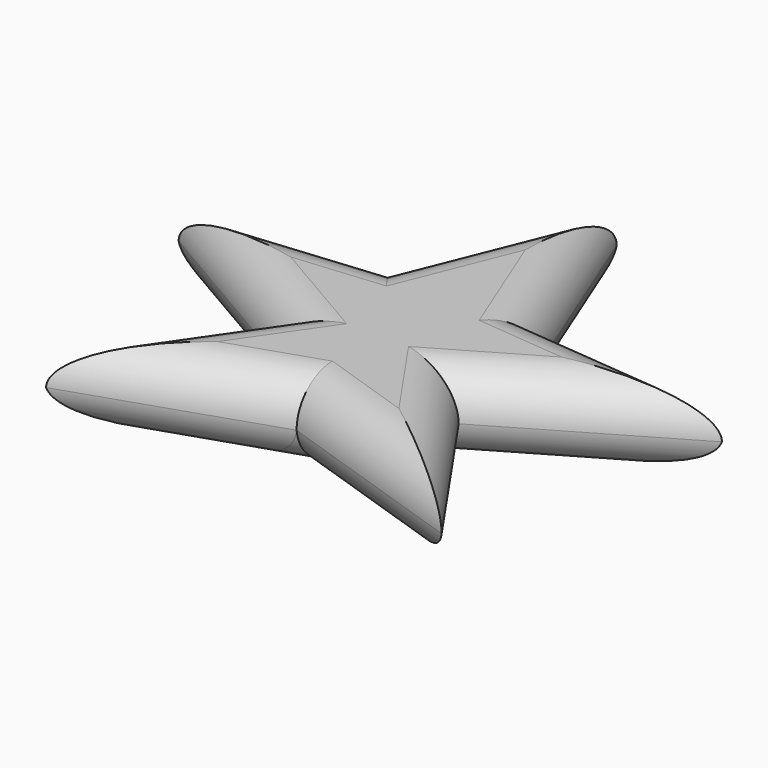
from build123d import *

# Parameters (mm, degrees)
F1_DEPTH      = 9.652
F2_R          = 5.08
F3_T4_DEPTH   = 48.7182027165
F3_T9_DEPTH   = 49.6907337444
F3_T14_DEPTH  = 49.6907337444
F3_T19_DEPTH  = 48.7182027165
F3_T24_DEPTH  = 50.0877618637
F3_T29_DEPTH  = 47.5225066811
F3_T34_DEPTH  = 50.1646809025
F3_T39_DEPTH  = 50.1646809025
F3_T44_DEPTH  = 47.5225066811
F3_T49_DEPTH  = 50.0877618637
F3_T55_DEPTH  = 49.6907337444
F3_T59_DEPTH  = 48.7182027165
F3_T66_DEPTH  = 49.6907337444
F3_T70_DEPTH  = 48.7182027165
F3_T77_DEPTH  = 50.0877618637
F3_T81_DEPTH  = 47.5225066811
F3_T88_DEPTH  = 50.1646809025
F3_T92_DEPTH  = 50.1646809025
F3_T99_DEPTH  = 47.5225066811
F3_T103_DEPTH = 50.0877618637


# Not quite as in the source:
# - a fillet or chamfer that OpenCascade refuses, or shapes differently, is made with other operations: its cross-section is extruded or revolved along the edge and cut away or added


with BuildPart() as f1:
    # F0 (on Top) → F1 (new body)
    with BuildSketch(Plane.XY):
        Polygon((9.0920295568, 17.9841070124), (0, 40.6463289496), (-9.0920295568, 17.9841070124), (-32.4367642404, 15.8125049123), (-10.9921818601, 3.3257867829), (-23.6146248879, -14.9971136204), (0, -7.1255727671), (23.6146248879, -14.9971136204), (10.9921818601, 3.3257867829), (32.4367642404, 15.8125049123), align=None)
    extrude(amount=F1_DEPTH)

    # F2
    f2_edges = [f1.edges().sort_by_distance(p)[0] for p in [
        (21.714473, 9.569146, 9.652),
        (17.303403, -5.835663, 9.652),
        (11.807312, -11.061343, 9.652),
        (-11.807312, -11.061343, 9.652),
        (-17.303403, -5.835663, 9.652),
        (-21.714473, 9.569146, 9.652),
        (-4.546015, 29.315218, 9.652),
        (4.546015, 29.315218, 9.652),
        (20.764397, 16.898306, 9.652),
        (-20.764397, 16.898306, 9.652),
    ]]
    fillet(f2_edges, radius=F2_R)

    # F3: fillet of radius 5.08 on 10 edges, made by hand


with BuildPart() as f3_tool2:
    # F3_s3 → F3_t4 (new body)
    with BuildSketch(Plane(origin=(43.2821955638, -4.026248662, 0), x_dir=(0, 0, 1), z_dir=(-0.9957012204, 0.0926233213, 0))):
        with BuildLine():
            ThreePointArc((4.572, 18.7489312754), (1.3125711686, 17.1021626927), (0, 13.6943950949))
            Line((0, 13.6943950949), (-0.1016, 13.6943950949))
            Line((-0.1016, 13.6943950949), (-0.1016, 18.7489312754))
            Line((-0.1016, 18.7489312754), (0, 18.8505312754))
            ThreePointArc((0, 18.8505312754), (2.286, 18.8505312754), (4.56184, 18.8500219991))
            Line((4.56184, 18.8500219991), (4.572, 18.7489312754))
        make_face()
    extrude(amount=F3_T4_DEPTH)

    split(bisect_by=Plane(origin=(14.046321235, 5.6353506813, 0), x_dir=(0, 0, 1), z_dir=(0.928092919, 0.3723486723, 0)), keep=Keep.TOP)


with BuildPart() as f1_1:
    add(f1.part)

    # F3_t1: cut F3_tool2
    add(f3_tool2.part, mode=Mode.SUBTRACT)


with BuildPart() as f3_tool7:
    # F3_s8 → F3_t9 (new body)
    with BuildSketch(Plane(origin=(-0.2491670879, 0.6210582369, 0), x_dir=(0, 0, 1), z_dir=(-0.3723486723, 0.928092919, 0))):
        with BuildLine():
            ThreePointArc((4.572, 15.1346066199), (1.3125711686, 13.4878380371), (0, 10.0800704394))
            Line((0, 10.0800704394), (-0.1016, 10.0800704394))
            Line((-0.1016, 10.0800704394), (-0.1016, 15.1346066199))
            Line((-0.1016, 15.1346066199), (0, 15.2362066199))
            ThreePointArc((0, 15.2362066199), (2.286, 15.2362066199), (4.56184, 15.2356973435))
            Line((4.56184, 15.2356973435), (4.572, 15.1346066199))
        make_face()
    extrude(amount=F3_T9_DEPTH)

    split(bisect_by=Plane(origin=(1.7365882856, 18.6683337526, 0), x_dir=(0, 0, 1), z_dir=(0.0926233213, 0.9957012204, 0)), keep=Keep.TOP)


with BuildPart() as f1_2:
    add(f1_1.part)

    # F3_t6: cut F3_tool7
    add(f3_tool7.part, mode=Mode.SUBTRACT)


with BuildPart() as f3_tool12:
    # F3_s13 → F3_t14 (new body)
    with BuildSketch(Plane(origin=(18.7514458253, 46.7386763625, 0), x_dir=(0, 0, 1), z_dir=(-0.3723486723, -0.928092919, 0))):
        with BuildLine():
            ThreePointArc((0, 10.0800704394), (1.3125711686, 13.4878380371), (4.572, 15.1346066199))
            Line((4.572, 15.1346066199), (4.56184, 15.2356973435))
            ThreePointArc((4.56184, 15.2356973435), (2.286, 15.2362066199), (0, 15.2362066199))
            Line((0, 15.2362066199), (-0.1016, 15.1346066199))
            Line((-0.1016, 15.1346066199), (-0.1016, 10.0800704394))
            Line((-0.1016, 10.0800704394), (0, 10.0800704394))
        make_face()
    extrude(amount=F3_T14_DEPTH)

    split(bisect_by=Plane(origin=(-1.7365882856, 18.6683337526, 0), x_dir=(0, 0, 1), z_dir=(-0.0926233213, 0.9957012204, 0)), keep=Keep.TOP)


with BuildPart() as f1_3:
    add(f1_2.part)

    # F3_t11: cut F3_tool12
    add(f3_tool12.part, mode=Mode.SUBTRACT)


with BuildPart() as f3_tool17:
    # F3_s18 → F3_t19 (new body)
    with BuildSketch(Plane(origin=(5.2265783378, 0.4861930816, 0), x_dir=(0, 0, 1), z_dir=(-0.9957012204, -0.0926233213, 0))):
        with BuildLine():
            ThreePointArc((0, 13.6943950949), (1.3125711686, 17.1021626927), (4.572, 18.7489312754))
            Line((4.572, 18.7489312754), (4.56184, 18.8500219991))
            ThreePointArc((4.56184, 18.8500219991), (2.286, 18.8505312754), (0, 18.8505312754))
            Line((0, 18.8505312754), (-0.1016, 18.7489312754))
            Line((-0.1016, 18.7489312754), (-0.1016, 13.6943950949))
            Line((-0.1016, 13.6943950949), (0, 13.6943950949))
        make_face()
    extrude(amount=F3_T19_DEPTH)

    split(bisect_by=Plane(origin=(-14.046321235, 5.6353506813, 0), x_dir=(0, 0, 1), z_dir=(-0.928092919, 0.3723486723, 0)), keep=Keep.TOP)


with BuildPart() as f1_4:
    add(f1_3.part)

    # F3_t16: cut F3_tool17
    add(f3_tool17.part, mode=Mode.SUBTRACT)


with BuildPart() as f3_tool22:
    # F3_s23 → F3_t24 (new body)
    with BuildSketch(Plane(origin=(-42.019750379, 24.4671950025, 0), x_dir=(0, 0, 1), z_dir=(0.8641753945, -0.5031907068, 0))):
        with BuildLine():
            ThreePointArc((0, -2.3974355258), (1.3125711686, 1.0103320719), (4.572, 2.6571006547))
            Line((4.572, 2.6571006547), (4.56184, 2.7581913783))
            ThreePointArc((4.56184, 2.7581913783), (2.286, 2.7587006547), (0, 2.7587006547))
            Line((0, 2.7587006547), (-0.1016, 2.6571006547))
            Line((-0.1016, 2.6571006547), (-0.1016, -2.3974355258))
            Line((-0.1016, -2.3974355258), (0, -2.3974355258))
        make_face()
    extrude(amount=F3_T24_DEPTH)

    split(bisect_by=Plane(origin=(-9.0082519421, 6.2056849307, 0), x_dir=(0, 0, 1), z_dir=(-0.8235075899, 0.5673052523, 0)), keep=Keep.TOP)


with BuildPart() as f1_5:
    add(f1_4.part)

    # F3_t21: cut F3_tool22
    add(f3_tool22.part, mode=Mode.SUBTRACT)


with BuildPart() as f3_tool27:
    # F3_s28 → F3_t29 (new body)
    with BuildSketch(Plane(origin=(5.1847323903, 7.5262241228, 0), x_dir=(0, 0, 1), z_dir=(-0.5673052523, -0.8235075899, 0))):
        with BuildLine():
            ThreePointArc((0, 5.8843453213), (1.3125711686, 9.292112919), (4.572, 10.9388815018))
            Line((4.572, 10.9388815018), (4.56184, 11.0399722254))
            ThreePointArc((4.56184, 11.0399722254), (2.286, 11.0404815018), (0, 11.0404815018))
            Line((0, 11.0404815018), (-0.1016, 10.9388815018))
            Line((-0.1016, 10.9388815018), (-0.1016, 5.8843453213))
            Line((-0.1016, 5.8843453213), (0, 5.8843453213))
        make_face()
    extrude(amount=F3_T29_DEPTH)

    split(bisect_by=Plane(origin=(-1.3370283566, -2.2962010066, 0), x_dir=(0, 0, 1), z_dir=(-0.5031907068, -0.8641753945, 0)), keep=Keep.TOP)


with BuildPart() as f1_6:
    add(f1_5.part)

    # F3_t26: cut F3_tool27
    add(f3_tool27.part, mode=Mode.SUBTRACT)


with BuildPart() as f3_tool32:
    # F3_s33 → F3_t34 (new body)
    with BuildSketch(Plane(origin=(-37.7401818022, -12.5800593605, 0), x_dir=(0, 0, 1), z_dir=(0.9486833074, 0.316227738, 0))):
        with BuildLine():
            ThreePointArc((0, 1.7053757593), (1.3125711686, 5.1131433571), (4.572, 6.7599119398))
            Line((4.572, 6.7599119398), (4.56184, 6.8610026635))
            ThreePointArc((4.56184, 6.8610026635), (2.286, 6.8615119398), (0, 6.8615119398))
            Line((0, 6.8615119398), (-0.1016, 6.7599119398))
            Line((-0.1016, 6.7599119398), (-0.1016, 1.7053757593))
            Line((-0.1016, 1.7053757593), (0, 1.7053757593))
        make_face()
    extrude(amount=F3_T34_DEPTH)

    split(bisect_by=Plane(origin=(-2.1376716615, -6.4130156168, 0), x_dir=(0, 0, 1), z_dir=(-0.316227738, -0.9486833074, 0)), keep=Keep.TOP)


with BuildPart() as f1_7:
    add(f1_6.part)

    # F3_t31: cut F3_tool32
    add(f3_tool32.part, mode=Mode.SUBTRACT)


with BuildPart() as f3_tool37:
    # F3_s38 → F3_t39 (new body)
    with BuildSketch(Plane(origin=(-9.8502135912, 3.2834042067, 0), x_dir=(0, 0, 1), z_dir=(0.9486833074, -0.316227738, 0))):
        with BuildLine():
            ThreePointArc((0, 1.7053757593), (1.3125711686, 5.1131433571), (4.572, 6.7599119398))
            Line((4.572, 6.7599119398), (4.56184, 6.8610026635))
            ThreePointArc((4.56184, 6.8610026635), (2.286, 6.8615119398), (0, 6.8615119398))
            Line((0, 6.8615119398), (-0.1016, 6.7599119398))
            Line((-0.1016, 6.7599119398), (-0.1016, 1.7053757593))
            Line((-0.1016, 1.7053757593), (0, 1.7053757593))
        make_face()
    extrude(amount=F3_T39_DEPTH)

    split(bisect_by=Plane(origin=(2.1376716615, -6.4130156168, 0), x_dir=(0, 0, 1), z_dir=(0.316227738, -0.9486833074, 0)), keep=Keep.TOP)


with BuildPart() as f1_8:
    add(f1_7.part)

    # F3_t36: cut F3_tool37
    add(f3_tool37.part, mode=Mode.SUBTRACT)


with BuildPart() as f3_tool42:
    # F3_s43 → F3_t44 (new body)
    with BuildSketch(Plane(origin=(21.7750352542, -31.6089208215, 0), x_dir=(0, 0, 1), z_dir=(-0.5673052523, 0.8235075899, 0))):
        with BuildLine():
            ThreePointArc((0, 5.8843453213), (1.3125711686, 9.292112919), (4.572, 10.9388815018))
            Line((4.572, 10.9388815018), (4.56184, 11.0399722254))
            ThreePointArc((4.56184, 11.0399722254), (2.286, 11.0404815018), (0, 11.0404815018))
            Line((0, 11.0404815018), (-0.1016, 10.9388815018))
            Line((-0.1016, 10.9388815018), (-0.1016, 5.8843453213))
            Line((-0.1016, 5.8843453213), (0, 5.8843453213))
        make_face()
    extrude(amount=F3_T44_DEPTH)

    split(bisect_by=Plane(origin=(1.3370283566, -2.2962010066, 0), x_dir=(0, 0, 1), z_dir=(0.5031907068, -0.8641753945, 0)), keep=Keep.TOP)


with BuildPart() as f1_9:
    add(f1_8.part)

    # F3_t41: cut F3_tool42
    add(f3_tool42.part, mode=Mode.SUBTRACT)


with BuildPart() as f3_tool47:
    # F3_s48 → F3_t49 (new body)
    with BuildSketch(Plane(origin=(-1.2648609916, -0.7365012941, 0), x_dir=(0, 0, 1), z_dir=(0.8641753945, 0.5031907068, 0))):
        with BuildLine():
            ThreePointArc((0, -2.3974355258), (1.3125711686, 1.0103320719), (4.572, 2.6571006547))
            Line((4.572, 2.6571006547), (4.56184, 2.7581913783))
            ThreePointArc((4.56184, 2.7581913783), (2.286, 2.7587006547), (0, 2.7587006547))
            Line((0, 2.7587006547), (-0.1016, 2.6571006547))
            Line((-0.1016, 2.6571006547), (-0.1016, -2.3974355258))
            Line((-0.1016, -2.3974355258), (0, -2.3974355258))
        make_face()
    extrude(amount=F3_T49_DEPTH)

    split(bisect_by=Plane(origin=(9.0082519421, 6.2056849307, 0), x_dir=(0, 0, 1), z_dir=(0.8235075899, 0.5673052523, 0)), keep=Keep.TOP)


with BuildPart() as f1_10:
    add(f1_9.part)

    # F3_t46: cut F3_tool47
    add(f3_tool47.part, mode=Mode.SUBTRACT)


with BuildPart() as f3_tool53:
    # F3_s54 → F3_t55 (new body)
    with BuildSketch(Plane(origin=(-0.2491670879, 0.6210582369, 0), x_dir=(0, 0, 1), z_dir=(-0.3723486723, 0.928092919, 0))):
        with BuildLine():
            ThreePointArc((4.572, 15.1346066199), (1.3125711686, 13.4878380371), (0, 10.0800704394))
            Line((0, 10.0800704394), (-0.1016, 10.0800704394))
            Line((-0.1016, 10.0800704394), (-0.1016, 15.1346066199))
            Line((-0.1016, 15.1346066199), (0, 15.2362066199))
            ThreePointArc((0, 15.2362066199), (2.286, 15.2362066199), (4.56184, 15.2356973435))
            Line((4.56184, 15.2356973435), (4.572, 15.1346066199))
        make_face()
    extrude(amount=F3_T55_DEPTH)

    split(bisect_by=Plane(origin=(1.7365882856, 18.6683337526, 0), x_dir=(0, 0, 1), z_dir=(-0.0926233213, -0.9957012204, 0)), keep=Keep.TOP)


with BuildPart() as f3_tool57:
    # F3_s58 → F3_t59 (new body)
    with BuildSketch(Plane(origin=(43.2821955638, -4.026248662, 0), x_dir=(0, 0, 1), z_dir=(-0.9957012204, 0.0926233213, 0))):
        with BuildLine():
            ThreePointArc((4.572, 18.7489312754), (1.3125711686, 17.1021626927), (0, 13.6943950949))
            Line((0, 13.6943950949), (-0.1016, 13.6943950949))
            Line((-0.1016, 13.6943950949), (-0.1016, 18.7489312754))
            Line((-0.1016, 18.7489312754), (0, 18.8505312754))
            ThreePointArc((0, 18.8505312754), (2.286, 18.8505312754), (4.56184, 18.8500219991))
            Line((4.56184, 18.8500219991), (4.572, 18.7489312754))
        make_face()
    extrude(amount=F3_T59_DEPTH)

    split(bisect_by=Plane(origin=(14.046321235, 5.6353506813, 0), x_dir=(0, 0, 1), z_dir=(-0.928092919, -0.3723486723, 0)), keep=Keep.TOP)


with BuildPart() as f3_tool53_1:
    add(f3_tool53.part)

    # F3_t61: intersect F3_tool57
    add(f3_tool57.part, mode=Mode.INTERSECT)


with BuildPart() as f1_11:
    add(f1_10.part)

    # F3_t51: cut F3_tool53
    add(f3_tool53_1.part, mode=Mode.SUBTRACT)


with BuildPart() as f3_tool64:
    # F3_s65 → F3_t66 (new body)
    with BuildSketch(Plane(origin=(18.7514458253, 46.7386763625, 0), x_dir=(0, 0, 1), z_dir=(-0.3723486723, -0.928092919, 0))):
        with BuildLine():
            ThreePointArc((0, 10.0800704394), (1.3125711686, 13.4878380371), (4.572, 15.1346066199))
            Line((4.572, 15.1346066199), (4.56184, 15.2356973435))
            ThreePointArc((4.56184, 15.2356973435), (2.286, 15.2362066199), (0, 15.2362066199))
            Line((0, 15.2362066199), (-0.1016, 15.1346066199))
            Line((-0.1016, 15.1346066199), (-0.1016, 10.0800704394))
            Line((-0.1016, 10.0800704394), (0, 10.0800704394))
        make_face()
    extrude(amount=F3_T66_DEPTH)

    split(bisect_by=Plane(origin=(-1.7365882856, 18.6683337526, 0), x_dir=(0, 0, 1), z_dir=(0.0926233213, -0.9957012204, 0)), keep=Keep.TOP)


with BuildPart() as f3_tool68:
    # F3_s69 → F3_t70 (new body)
    with BuildSketch(Plane(origin=(5.2265783378, 0.4861930816, 0), x_dir=(0, 0, 1), z_dir=(-0.9957012204, -0.0926233213, 0))):
        with BuildLine():
            ThreePointArc((0, 13.6943950949), (1.3125711686, 17.1021626927), (4.572, 18.7489312754))
            Line((4.572, 18.7489312754), (4.56184, 18.8500219991))
            ThreePointArc((4.56184, 18.8500219991), (2.286, 18.8505312754), (0, 18.8505312754))
            Line((0, 18.8505312754), (-0.1016, 18.7489312754))
            Line((-0.1016, 18.7489312754), (-0.1016, 13.6943950949))
            Line((-0.1016, 13.6943950949), (0, 13.6943950949))
        make_face()
    extrude(amount=F3_T70_DEPTH)

    split(bisect_by=Plane(origin=(-14.046321235, 5.6353506813, 0), x_dir=(0, 0, 1), z_dir=(0.928092919, -0.3723486723, 0)), keep=Keep.TOP)


with BuildPart() as f3_tool64_1:
    add(f3_tool64.part)

    # F3_t72: intersect F3_tool68
    add(f3_tool68.part, mode=Mode.INTERSECT)


with BuildPart() as f1_12:
    add(f1_11.part)

    # F3_t62: cut F3_tool64
    add(f3_tool64_1.part, mode=Mode.SUBTRACT)


with BuildPart() as f3_tool75:
    # F3_s76 → F3_t77 (new body)
    with BuildSketch(Plane(origin=(-42.019750379, 24.4671950025, 0), x_dir=(0, 0, 1), z_dir=(0.8641753945, -0.5031907068, 0))):
        with BuildLine():
            ThreePointArc((0, -2.3974355258), (1.3125711686, 1.0103320719), (4.572, 2.6571006547))
            Line((4.572, 2.6571006547), (4.56184, 2.7581913783))
            ThreePointArc((4.56184, 2.7581913783), (2.286, 2.7587006547), (0, 2.7587006547))
            Line((0, 2.7587006547), (-0.1016, 2.6571006547))
            Line((-0.1016, 2.6571006547), (-0.1016, -2.3974355258))
            Line((-0.1016, -2.3974355258), (0, -2.3974355258))
        make_face()
    extrude(amount=F3_T77_DEPTH)

    split(bisect_by=Plane(origin=(-9.0082519421, 6.2056849307, 0), x_dir=(0, 0, 1), z_dir=(0.8235075899, -0.5673052523, 0)), keep=Keep.TOP)


with BuildPart() as f3_tool79:
    # F3_s80 → F3_t81 (new body)
    with BuildSketch(Plane(origin=(5.1847323903, 7.5262241228, 0), x_dir=(0, 0, 1), z_dir=(-0.5673052523, -0.8235075899, 0))):
        with BuildLine():
            ThreePointArc((0, 5.8843453213), (1.3125711686, 9.292112919), (4.572, 10.9388815018))
            Line((4.572, 10.9388815018), (4.56184, 11.0399722254))
            ThreePointArc((4.56184, 11.0399722254), (2.286, 11.0404815018), (0, 11.0404815018))
            Line((0, 11.0404815018), (-0.1016, 10.9388815018))
            Line((-0.1016, 10.9388815018), (-0.1016, 5.8843453213))
            Line((-0.1016, 5.8843453213), (0, 5.8843453213))
        make_face()
    extrude(amount=F3_T81_DEPTH)

    split(bisect_by=Plane(origin=(-1.3370283566, -2.2962010066, 0), x_dir=(0, 0, 1), z_dir=(0.5031907068, 0.8641753945, 0)), keep=Keep.TOP)


with BuildPart() as f3_tool75_1:
    add(f3_tool75.part)

    # F3_t83: intersect F3_tool79
    add(f3_tool79.part, mode=Mode.INTERSECT)


with BuildPart() as f1_13:
    add(f1_12.part)

    # F3_t73: cut F3_tool75
    add(f3_tool75_1.part, mode=Mode.SUBTRACT)


with BuildPart() as f3_tool86:
    # F3_s87 → F3_t88 (new body)
    with BuildSketch(Plane(origin=(-37.7401818022, -12.5800593605, 0), x_dir=(0, 0, 1), z_dir=(0.9486833074, 0.316227738, 0))):
        with BuildLine():
            ThreePointArc((0, 1.7053757593), (1.3125711686, 5.1131433571), (4.572, 6.7599119398))
            Line((4.572, 6.7599119398), (4.56184, 6.8610026635))
            ThreePointArc((4.56184, 6.8610026635), (2.286, 6.8615119398), (0, 6.8615119398))
            Line((0, 6.8615119398), (-0.1016, 6.7599119398))
            Line((-0.1016, 6.7599119398), (-0.1016, 1.7053757593))
            Line((-0.1016, 1.7053757593), (0, 1.7053757593))
        make_face()
    extrude(amount=F3_T88_DEPTH)

    split(bisect_by=Plane(origin=(-2.1376716615, -6.4130156168, 0), x_dir=(0, 0, 1), z_dir=(0.316227738, 0.9486833074, 0)), keep=Keep.TOP)


with BuildPart() as f3_tool90:
    # F3_s91 → F3_t92 (new body)
    with BuildSketch(Plane(origin=(-9.8502135912, 3.2834042067, 0), x_dir=(0, 0, 1), z_dir=(0.9486833074, -0.316227738, 0))):
        with BuildLine():
            ThreePointArc((0, 1.7053757593), (1.3125711686, 5.1131433571), (4.572, 6.7599119398))
            Line((4.572, 6.7599119398), (4.56184, 6.8610026635))
            ThreePointArc((4.56184, 6.8610026635), (2.286, 6.8615119398), (0, 6.8615119398))
            Line((0, 6.8615119398), (-0.1016, 6.7599119398))
            Line((-0.1016, 6.7599119398), (-0.1016, 1.7053757593))
            Line((-0.1016, 1.7053757593), (0, 1.7053757593))
        make_face()
    extrude(amount=F3_T92_DEPTH)

    split(bisect_by=Plane(origin=(2.1376716615, -6.4130156168, 0), x_dir=(0, 0, 1), z_dir=(-0.316227738, 0.9486833074, 0)), keep=Keep.TOP)


with BuildPart() as f3_tool86_1:
    add(f3_tool86.part)

    # F3_t94: intersect F3_tool90
    add(f3_tool90.part, mode=Mode.INTERSECT)


with BuildPart() as f1_14:
    add(f1_13.part)

    # F3_t84: cut F3_tool86
    add(f3_tool86_1.part, mode=Mode.SUBTRACT)


with BuildPart() as f3_tool97:
    # F3_s98 → F3_t99 (new body)
    with BuildSketch(Plane(origin=(21.7750352542, -31.6089208215, 0), x_dir=(0, 0, 1), z_dir=(-0.5673052523, 0.8235075899, 0))):
        with BuildLine():
            ThreePointArc((0, 5.8843453213), (1.3125711686, 9.292112919), (4.572, 10.9388815018))
            Line((4.572, 10.9388815018), (4.56184, 11.0399722254))
            ThreePointArc((4.56184, 11.0399722254), (2.286, 11.0404815018), (0, 11.0404815018))
            Line((0, 11.0404815018), (-0.1016, 10.9388815018))
            Line((-0.1016, 10.9388815018), (-0.1016, 5.8843453213))
            Line((-0.1016, 5.8843453213), (0, 5.8843453213))
        make_face()
    extrude(amount=F3_T99_DEPTH)

    split(bisect_by=Plane(origin=(1.3370283566, -2.2962010066, 0), x_dir=(0, 0, 1), z_dir=(-0.5031907068, 0.8641753945, 0)), keep=Keep.TOP)


with BuildPart() as f3_tool101:
    # F3_s102 → F3_t103 (new body)
    with BuildSketch(Plane(origin=(-1.2648609916, -0.7365012941, 0), x_dir=(0, 0, 1), z_dir=(0.8641753945, 0.5031907068, 0))):
        with BuildLine():
            ThreePointArc((0, -2.3974355258), (1.3125711686, 1.0103320719), (4.572, 2.6571006547))
            Line((4.572, 2.6571006547), (4.56184, 2.7581913783))
            ThreePointArc((4.56184, 2.7581913783), (2.286, 2.7587006547), (0, 2.7587006547))
            Line((0, 2.7587006547), (-0.1016, 2.6571006547))
            Line((-0.1016, 2.6571006547), (-0.1016, -2.3974355258))
            Line((-0.1016, -2.3974355258), (0, -2.3974355258))
        make_face()
    extrude(amount=F3_T103_DEPTH)

    split(bisect_by=Plane(origin=(9.0082519421, 6.2056849307, 0), x_dir=(0, 0, 1), z_dir=(-0.8235075899, -0.5673052523, 0)), keep=Keep.TOP)


with BuildPart() as f3_tool97_1:
    add(f3_tool97.part)

    # F3_t105: intersect F3_tool101
    add(f3_tool101.part, mode=Mode.INTERSECT)


with BuildPart() as f1_15:
    add(f1_14.part)

    # F3_t95: cut F3_tool97
    add(f3_tool97_1.part, mode=Mode.SUBTRACT)


solid = f1_15.part
